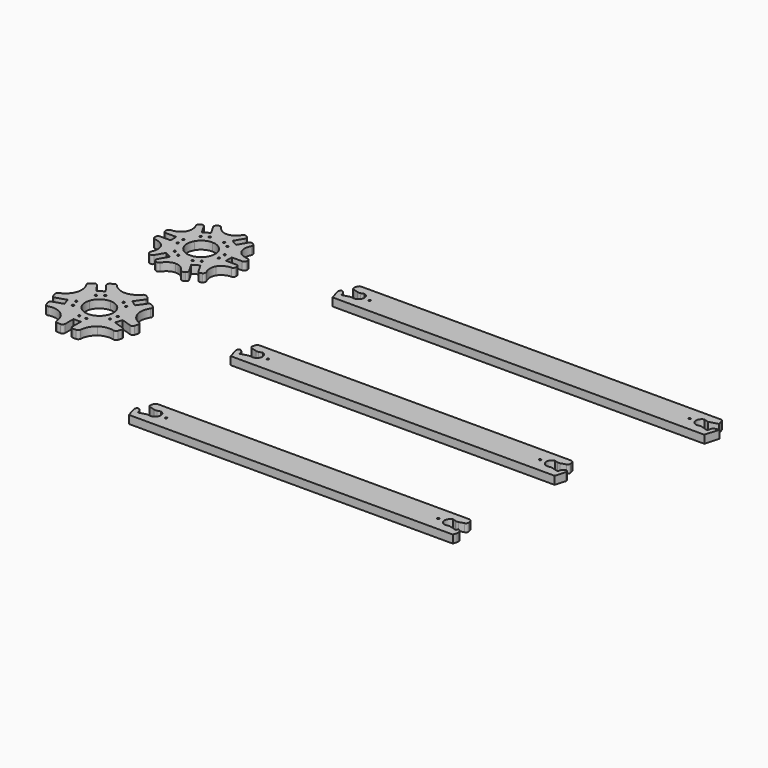
from build123d import *

# Parameters (mm, degrees)
F1_R         = 0.4
F2_DEPTH     = 3.15
F4_COUNT     = 6
F4_ANGLE     = 300
F5_R         = 0.4
F6_DEPTH     = 3.15
F9_COUNT     = 5
F9_ANGLE     = 288
F10_R        = 0.4
F11_DEPTH    = 3.15
F12_R        = 2
F13_T1_DEPTH = 11.2423560541
F13_T3_DEPTH = 8.15
F13_T5_DEPTH = 6.9177702505
F14_R        = 0.4
F15_DEPTH    = 3.15
F16_R        = 2
F17_T1_DEPTH = 6.9177702505
F17_T3_DEPTH = 8.15
F17_T5_DEPTH = 11.2423560541
F18_R        = 0.4
F19_DEPTH    = 3.15
F20_T1_DEPTH = 6.0174538576
F20_T3_DEPTH = 8.6930905145
F20_T5_DEPTH = 13.1438739724
F21_T1_DEPTH = 6.9177702505
F21_T3_DEPTH = 8.15
F21_T5_DEPTH = 11.2423560542


# Not quite as in the source:
# - a fillet or chamfer that OpenCascade refuses, or shapes differently, is made with other operations: its cross-section is extruded or revolved along the edge and cut away or added
# - a feature names something its author has since deleted; it is built from what else it names


with BuildPart() as f2:
    # F1 (on Top) → F2 (new body)
    with BuildSketch(Plane.XY):
        with BuildLine():
            ThreePointArc((0, 5.5), (2.75, 4.7631397208), (4.7631397208, 2.75))
            Line((4.7631397208, 2.75), (9.4396769013, 5.45))
            Line((9.4396769013, 5.45), (10.8253175473, 6.25))
            add(Edge.make_bspline(
                [(10.9160447626, 11.090214333), (9.5815334772, 8.4042972031), (10.8253175473, 6.25)],
                knots=[5.4423529264, 5.4423529264, 5.4423529264, 6.2831853072, 6.2831853072, 6.2831853072], degree=2, weights=[1, 0.9129191552, 1]))
            ThreePointArc((10.9160447626, 11.090214333), (10.9778655219, 11.8240320404), (10.5204937972, 12.4011986882))
            Line((10.5204937972, 12.4011986882), (10.1001116042, 12.6439064606))
            ThreePointArc((10.1001116042, 12.6439064606), (9.3412925591, 12.7438068831), (8.7340862004, 12.2778810568))
            Line((8.7340862004, 12.2778810568), (6.6840862004, 8.7271769013))
            Line((6.6840862004, 8.7271769013), (5.45, 9.4396769013))
            Line((5.45, 9.4396769013), (4.2159137996, 10.1521769013))
            Line((4.2159137996, 10.1521769013), (6.2659137996, 13.7028810568))
            ThreePointArc((6.2659137996, 13.7028810568), (6.3658142221, 14.4617001019), (5.8998883958, 15.0689064606))
            Line((5.8998883958, 15.0689064606), (5.4795062028, 15.3116142329))
            ThreePointArc((5.4795062028, 15.3116142329), (4.7509793612, 15.4191264414), (4.1463849645, 14.9986792397))
            add(Edge.make_bspline(
                [(0, 12.5), (2.4875681402, 12.5), (4.1463849645, 14.9986792397)],
                knots=[0, 0, 0, 0.8408323808, 0.8408323808, 0.8408323808], degree=2, weights=[1, 0.9129191552, 1]))
            Line((0, 12.5), (0, 10.9))
            Line((0, 10.9), (0, 5.5))
        make_face()
        with Locations((5.2871339923, 6.307584701)):
            Circle(F1_R, mode=Mode.SUBTRACT)
        with Locations((2.8189615915, 7.732584701)):
            Circle(F1_R, mode=Mode.SUBTRACT)
    extrude(amount=F2_DEPTH)

    # F4: F2 ×6 about axis
    f4_axis = Axis((0, 0, 10), (0, 0, -1))


with BuildPart() as f2_1:
    add(f2.part)
    for i in range(1, F4_COUNT):
        add(f2.part.rotate(f4_axis, i * F4_ANGLE / (F4_COUNT - 1)))


with BuildPart() as f6:
    # F5 (on Top) → F6 (new body)
    with BuildSketch(Plane.XY):
        with BuildLine():
            ThreePointArc((0, -44.5), (3.2328188876, -45.5504065309), (5.2308108396, -48.3004065309))
            Line((5.2308108396, -48.3004065309), (10.3665160276, -46.6317147613))
            Line((10.3665160276, -46.6317147613), (11.8882064537, -46.1372875703))
            add(Edge.make_bspline(
                [(12.6600498513, -40.5786625801), (10.9558427712, -43.267767214), (11.8882064537, -46.1372875703)],
                knots=[5.4507768063, 5.4507768063, 5.4507768063, 6.2831853072, 6.2831853072, 6.2831853072], degree=2, weights=[1, 0.9146301154, 1]))
            ThreePointArc((12.6600498513, -40.5786625801), (12.797616851, -39.8556747592), (12.4031733071, -39.2343452499))
            Line((12.4031733071, -39.2343452499), (11.366430248, -38.4811073268))
            ThreePointArc((11.366430248, -38.4811073268), (10.6222105307, -38.3024359806), (9.9696280014, -38.7023390689))
            Line((9.9696280014, -38.7023390689), (7.559708467, -42.0193087458))
            Line((7.559708467, -42.0193087458), (6.40685925, -41.1817147613))
            Line((6.40685925, -41.1817147613), (5.254010033, -40.3441207768))
            Line((5.254010033, -40.3441207768), (7.6639295674, -37.0271510999))
            ThreePointArc((7.6639295674, -37.0271510999), (7.8426009136, -36.2829313825), (7.4426978253, -35.6303488532))
            Line((7.4426978253, -35.6303488532), (6.4059547662, -34.8771109302))
            ThreePointArc((6.4059547662, -34.8771109302), (5.6931455292, -34.693974205), (5.0480537917, -35.0482237198))
            add(Edge.make_bspline(
                [(0, -37.5), (3.0171922563, -37.5), (5.0480537917, -35.0482237198)],
                knots=[0, 0, 0, 0.8324085009, 0.8324085009, 0.8324085009], degree=2, weights=[1, 0.9146301154, 1]))
            Line((0, -37.5), (0, -39.1))
            Line((0, -39.1), (0, -44.5))
        make_face()
        with Locations((5.9174926548, -44.2796248992)):
            Circle(F5_R, mode=Mode.SUBTRACT)
        with Locations((3.6117942208, -42.6044369302)):
            Circle(F5_R, mode=Mode.SUBTRACT)
    extrude(amount=F6_DEPTH)

    # F9: F6 ×5 about axis
    f9_axis = Axis((0, -50, 25), (0, 0, 1))


with BuildPart() as f6_1:
    add(f6.part)
    for i in range(1, F9_COUNT):
        add(f6.part.rotate(f9_axis, i * F9_ANGLE / (F9_COUNT - 1)))


with BuildPart() as f11:
    # F10 (on Top) → F11 (new body)
    with BuildSketch(Plane.XY):
        with BuildLine():
            Line((50, 5.55), (51.591436891, 0))
            Line((51.591436891, 0), (197.708563109, 0))
            Line((197.708563109, 0), (199.3, 5.55))
            Line((199.3, 5.55), (197.1123413707, 4.9226989824))
            Line((197.1123413707, 4.9226989824), (196.5317412663, 2.8979057922))
            Line((196.5317412663, 2.8979057922), (193.2913948098, 3.8270601869))
            Line((193.2913948098, 3.8270601869), (192.6927821889, 3.65541078))
            ThreePointArc((192.6927821889, 3.65541078), (189.9120802217, 5.1700720177), (191.4267414594, 7.9507739849))
            Line((191.4267414594, 7.9507739849), (193.2913948098, 7.4160932406))
            Line((193.2913948098, 7.4160932406), (196.8, 8.4221695893))
            Line((196.8, 8.4221695893), (196.0321444859, 11.1))
            Line((196.0321444859, 11.1), (53.2678555141, 11.1))
            Line((53.2678555141, 11.1), (52.5, 8.4221695893))
            Line((52.5, 8.4221695893), (56.0086051902, 7.4160932406))
            Line((56.0086051902, 7.4160932406), (57.8732585406, 7.9507739849))
            ThreePointArc((57.8732585406, 7.9507739849), (59.3879197783, 5.1700720177), (56.6072178111, 3.65541078))
            Line((56.6072178111, 3.65541078), (56.0086051902, 3.8270601869))
            Line((56.0086051902, 3.8270601869), (52.7682587337, 2.8979057922))
            Line((52.7682587337, 2.8979057922), (52.1876586293, 4.9226989824))
            Line((52.1876586293, 4.9226989824), (50, 5.55))
        make_face()
        with Locations((61.7649168703, 5.55)):
            Circle(F10_R, mode=Mode.SUBTRACT)
        with Locations((187.5350831297, 5.55)):
            Circle(F10_R, mode=Mode.SUBTRACT)
    extrude(amount=F11_DEPTH)

    # F12
    f12_edges = [f11.edges().sort_by_distance(p)[0] for p in [
        (56.008605, 7.416093, 1.575),
        (56.008605, 3.82706, 1.575),
        (52.187659, 4.922699, 1.575),
    ]]
    fillet(f12_edges, radius=F12_R)

    # F13: fillet of radius 1 on 4 edges, made by hand

    # F13_s2 → F13_t1 (cut)
    with BuildSketch(Plane.XY.offset(-4.046178027)):
        with BuildLine():
            ThreePointArc((51.1219865116, 5.2282755449), (50.5303023465, 4.7502246957), (50.446111125, 3.9942256191))
            Line((50.446111125, 3.9942256191), (50, 5.55))
            Line((50, 5.55), (51.1219865116, 5.2282755449))
        make_face()
    extrude(amount=F13_T1_DEPTH, mode=Mode.SUBTRACT)

    # F13_s4 → F13_t3 (cut)
    with BuildSketch(Plane.XY.offset(-2.5)):
        with BuildLine():
            ThreePointArc((53.4612616959, 8.1465322335), (52.8622793446, 8.6229843092), (52.7756373558, 9.3834312853))
            Line((52.7756373558, 9.3834312853), (52.5, 8.4221695893))
            Line((52.5, 8.4221695893), (53.4612616959, 8.1465322335))
        make_face()
    extrude(amount=F13_T3_DEPTH, mode=Mode.SUBTRACT)

    # F13_s6 → F13_t5 (cut)
    with BuildSketch(Plane.XY.offset(-1.8838851253)):
        with BuildLine():
            ThreePointArc((53.0601478683, 10.3756373558), (53.4195945411, 10.89863551), (54.0214095642, 11.1))
            Line((54.0214095642, 11.1), (53.2678555141, 11.1))
            Line((53.2678555141, 11.1), (53.0601478683, 10.3756373558))
        make_face()
        with BuildLine():
            ThreePointArc((195.2785904358, 11.1), (195.8804054589, 10.89863551), (196.2398521317, 10.3756373558))
            Line((196.2398521317, 10.3756373558), (196.0321444859, 11.1))
            Line((196.0321444859, 11.1), (195.2785904358, 11.1))
        make_face()
    extrude(amount=F13_T5_DEPTH, mode=Mode.SUBTRACT)


with BuildPart() as f15:
    # F14 (on Top) → F15 (new body)
    with BuildSketch(Plane.XY):
        with BuildLine():
            Line((50, -44.45), (51.591436891, -50))
            Line((51.591436891, -50), (178.908563109, -50))
            Line((178.908563109, -50), (180.5, -44.45))
            Line((180.5, -44.45), (178.3123413707, -45.0773010176))
            Line((178.3123413707, -45.0773010176), (177.7317412663, -47.1020942078))
            Line((177.7317412663, -47.1020942078), (174.4913948098, -46.1729398131))
            Line((174.4913948098, -46.1729398131), (173.8927821889, -46.34458922))
            ThreePointArc((173.8927821889, -46.34458922), (171.1120802217, -44.8299279823), (172.6267414594, -42.0492260151))
            Line((172.6267414594, -42.0492260151), (174.4913948098, -42.5839067594))
            Line((174.4913948098, -42.5839067594), (178, -41.5778304107))
            Line((178, -41.5778304107), (177.2321444859, -38.9))
            Line((177.2321444859, -38.9), (53.2678555141, -38.9))
            Line((53.2678555141, -38.9), (52.5, -41.5778304107))
            Line((52.5, -41.5778304107), (56.0086051902, -42.5839067594))
            Line((56.0086051902, -42.5839067594), (57.8732585406, -42.0492260151))
            ThreePointArc((57.8732585406, -42.0492260151), (59.3879197783, -44.8299279823), (56.6072178111, -46.34458922))
            Line((56.6072178111, -46.34458922), (56.0086051902, -46.1729398131))
            Line((56.0086051902, -46.1729398131), (52.7682587337, -47.1020942078))
            Line((52.7682587337, -47.1020942078), (52.1876586293, -45.0773010176))
            Line((52.1876586293, -45.0773010176), (50, -44.45))
        make_face()
        with Locations((61.7649168703, -44.45)):
            Circle(F14_R, mode=Mode.SUBTRACT)
        with Locations((168.7350831297, -44.45)):
            Circle(F14_R, mode=Mode.SUBTRACT)
    extrude(amount=F15_DEPTH)

    # F16
    f16_edges = [f15.edges().sort_by_distance(p)[0] for p in [
        (52.187659, -45.077301, 1.575),
        (56.008605, -46.17294, 1.575),
        (56.008605, -42.583907, 1.575),
        (174.491395, -42.583907, 1.575),
        (174.491395, -46.17294, 1.575),
        (178.312341, -45.077301, 1.575),
    ]]
    fillet(f16_edges, radius=F16_R)

    # F17: fillet of radius 1 on 6 edges, made by hand

    # F17_s2 → F17_t1 (cut)
    with BuildSketch(Plane.XY.offset(-1.8838851253)):
        with BuildLine():
            ThreePointArc((176.4785904358, -38.9), (177.0804054589, -39.10136449), (177.4398521317, -39.6243626442))
            Line((177.4398521317, -39.6243626442), (177.2321444859, -38.9))
            Line((177.2321444859, -38.9), (176.4785904358, -38.9))
        make_face()
        with BuildLine():
            ThreePointArc((53.0601478683, -39.6243626442), (53.4195945411, -39.10136449), (54.0214095642, -38.9))
            Line((54.0214095642, -38.9), (53.2678555141, -38.9))
            Line((53.2678555141, -38.9), (53.0601478683, -39.6243626442))
        make_face()
    extrude(amount=F17_T1_DEPTH, mode=Mode.SUBTRACT)

    # F17_s4 → F17_t3 (cut)
    with BuildSketch(Plane.XY.offset(-2.5)):
        with BuildLine():
            ThreePointArc((177.7243626442, -40.6165687147), (177.6377206554, -41.3770156908), (177.0387383041, -41.8534677665))
            Line((177.0387383041, -41.8534677665), (178, -41.5778304107))
            Line((178, -41.5778304107), (177.7243626442, -40.6165687147))
        make_face()
        with BuildLine():
            ThreePointArc((53.4612616959, -41.8534677665), (52.8622793446, -41.3770156908), (52.7756373558, -40.6165687147))
            Line((52.7756373558, -40.6165687147), (52.5, -41.5778304107))
            Line((52.5, -41.5778304107), (53.4612616959, -41.8534677665))
        make_face()
    extrude(amount=F17_T3_DEPTH, mode=Mode.SUBTRACT)

    # F17_s6 → F17_t5 (cut)
    with BuildSketch(Plane.XY.offset(-4.046178027)):
        with BuildLine():
            ThreePointArc((180.053888875, -46.0057743809), (179.9696976535, -45.2497753043), (179.3780134884, -44.7717244551))
            Line((179.3780134884, -44.7717244551), (180.5, -44.45))
            Line((180.5, -44.45), (180.053888875, -46.0057743809))
        make_face()
        with BuildLine():
            ThreePointArc((51.1219865116, -44.7717244551), (50.5303023465, -45.2497753043), (50.446111125, -46.0057743809))
            Line((50.446111125, -46.0057743809), (50, -44.45))
            Line((50, -44.45), (51.1219865116, -44.7717244551))
        make_face()
    extrude(amount=F17_T5_DEPTH, mode=Mode.SUBTRACT)


with BuildPart() as f19:
    # F18 (on Top) → F19 (new body)
    with BuildSketch(Plane.XY):
        with BuildLine():
            Line((50, -94.45), (51.591436891, -100))
            Line((51.591436891, -100), (178.908563109, -100))
            Line((178.908563109, -100), (179.8772810541, -96.6216790463))
            Line((179.8772810541, -96.6216790463), (178.0220413185, -96.0896976127))
            Line((178.0220413185, -96.0896976127), (177.7317412663, -97.1020942078))
            Line((177.7317412663, -97.1020942078), (174.4913948098, -96.1729398131))
            Line((174.4913948098, -96.1729398131), (173.8927821889, -96.34458922))
            ThreePointArc((173.8927821889, -96.34458922), (171.1120802217, -94.8299279823), (172.6267414594, -92.0492260151))
            Line((172.6267414594, -92.0492260151), (174.4913948098, -92.5839067594))
            Line((174.4913948098, -92.5839067594), (178, -91.5778304107))
            Line((178, -91.5778304107), (177.2321444859, -88.9))
            Line((177.2321444859, -88.9), (53.2678555141, -88.9))
            Line((53.2678555141, -88.9), (52.5, -91.5778304107))
            Line((52.5, -91.5778304107), (56.0086051902, -92.5839067594))
            Line((56.0086051902, -92.5839067594), (57.8732585406, -92.0492260151))
            ThreePointArc((57.8732585406, -92.0492260151), (59.3879197783, -94.8299279823), (56.6072178111, -96.34458922))
            Line((56.6072178111, -96.34458922), (56.0086051902, -96.1729398131))
            Line((56.0086051902, -96.1729398131), (52.7682587337, -97.1020942078))
            Line((52.7682587337, -97.1020942078), (52.1876586293, -95.0773010176))
            Line((52.1876586293, -95.0773010176), (50, -94.45))
        make_face()
        with Locations((61.7649168703, -94.45)):
            Circle(F18_R, mode=Mode.SUBTRACT)
        with Locations((168.7350831297, -94.45)):
            Circle(F18_R, mode=Mode.SUBTRACT)
    extrude(amount=F19_DEPTH)

    # F20: fillet of radius 2 on 6 edges, made by hand

    # F20_s2 → F20_t1 (cut)
    with BuildSketch(Plane.XY.offset(-1.4337269288)):
        with BuildLine():
            ThreePointArc((175.0426695215, -96.331015293), (174.4913948098, -96.2535386849), (173.9401200982, -96.331015293))
            Line((173.9401200982, -96.331015293), (174.4913948098, -96.1729398131))
            Line((174.4913948098, -96.1729398131), (175.0426695215, -96.331015293))
        make_face()
        with BuildLine():
            ThreePointArc((173.9401200982, -92.4258312796), (174.4913948098, -92.5033078877), (175.0426695215, -92.4258312796))
            Line((175.0426695215, -92.4258312796), (174.4913948098, -92.5839067594))
            Line((174.4913948098, -92.5839067594), (173.9401200982, -92.4258312796))
        make_face()
        with BuildLine():
            ThreePointArc((55.4573304785, -92.4258312796), (56.0086051902, -92.5033078877), (56.5598799018, -92.4258312796))
            Line((56.5598799018, -92.4258312796), (56.0086051902, -92.5839067594))
            Line((56.0086051902, -92.5839067594), (55.4573304785, -92.4258312796))
        make_face()
        with BuildLine():
            ThreePointArc((56.5598799018, -96.331015293), (56.0086051902, -96.2535386849), (55.4573304785, -96.331015293))
            Line((55.4573304785, -96.331015293), (56.0086051902, -96.1729398131))
            Line((56.0086051902, -96.1729398131), (56.5598799018, -96.331015293))
        make_face()
    extrude(amount=F20_T1_DEPTH, mode=Mode.SUBTRACT)

    # F20_s4 → F20_t3 (cut)
    with BuildSketch(Plane.XY.offset(-2.7715452573)):
        with BuildLine():
            ThreePointArc((51.1219865116, -94.7717244551), (51.9849253623, -95.2800342846), (52.4932351918, -96.1429731353))
            Line((52.4932351918, -96.1429731353), (52.1876586293, -95.0773010176))
            Line((52.1876586293, -95.0773010176), (51.1219865116, -94.7717244551))
        make_face()
    extrude(amount=F20_T3_DEPTH, mode=Mode.SUBTRACT)

    # F20_s6 → F20_t5 (cut)
    with BuildSketch(Plane.XY.offset(-4.9969369862)):
        with BuildLine():
            ThreePointArc((179.3263440549, -98.5430246951), (179.1697619196, -97.0528935098), (178.0220413185, -96.0896976127))
            Line((178.0220413185, -96.0896976127), (179.8772810541, -96.6216790463))
            Line((179.8772810541, -96.6216790463), (179.3263440549, -98.5430246951))
        make_face()
    extrude(amount=F20_T5_DEPTH, mode=Mode.SUBTRACT)

    # F21: fillet of radius 1 on 5 edges, made by hand

    # F21_s2 → F21_t1 (cut)
    with BuildSketch(Plane.XY.offset(-1.8838851253)):
        with BuildLine():
            ThreePointArc((176.4785904358, -88.9), (177.0804054589, -89.10136449), (177.4398521317, -89.6243626442))
            Line((177.4398521317, -89.6243626442), (177.2321444859, -88.9))
            Line((177.2321444859, -88.9), (176.4785904358, -88.9))
        make_face()
        with BuildLine():
            ThreePointArc((53.0601478683, -89.6243626442), (53.4195945411, -89.10136449), (54.0214095642, -88.9))
            Line((54.0214095642, -88.9), (53.2678555141, -88.9))
            Line((53.2678555141, -88.9), (53.0601478683, -89.6243626442))
        make_face()
    extrude(amount=F21_T1_DEPTH, mode=Mode.SUBTRACT)

    # F21_s4 → F21_t3 (cut)
    with BuildSketch(Plane.XY.offset(-2.5)):
        with BuildLine():
            ThreePointArc((177.7243626442, -90.6165687147), (177.6377206554, -91.3770156908), (177.0387383041, -91.8534677665))
            Line((177.0387383041, -91.8534677665), (178, -91.5778304107))
            Line((178, -91.5778304107), (177.7243626442, -90.6165687147))
        make_face()
        with BuildLine():
            ThreePointArc((53.4612616959, -91.8534677665), (52.8622793446, -91.3770156908), (52.7756373558, -90.6165687147))
            Line((52.7756373558, -90.6165687147), (52.5, -91.5778304107))
            Line((52.5, -91.5778304107), (53.4612616959, -91.8534677665))
        make_face()
    extrude(amount=F21_T3_DEPTH, mode=Mode.SUBTRACT)

    # F21_s6 → F21_t5 (cut)
    with BuildSketch(Plane.XY.offset(-4.0461780271)):
        with BuildLine():
            ThreePointArc((51.1219865116, -94.7717244551), (50.5303023465, -95.2497753043), (50.446111125, -96.005774381))
            Line((50.446111125, -96.005774381), (50, -94.45))
            Line((50, -94.45), (51.1219865116, -94.7717244551))
        make_face()
    extrude(amount=F21_T5_DEPTH, mode=Mode.SUBTRACT)


solid = Compound([f2_1.part, f6_1.part, f11.part, f15.part, f19.part])
